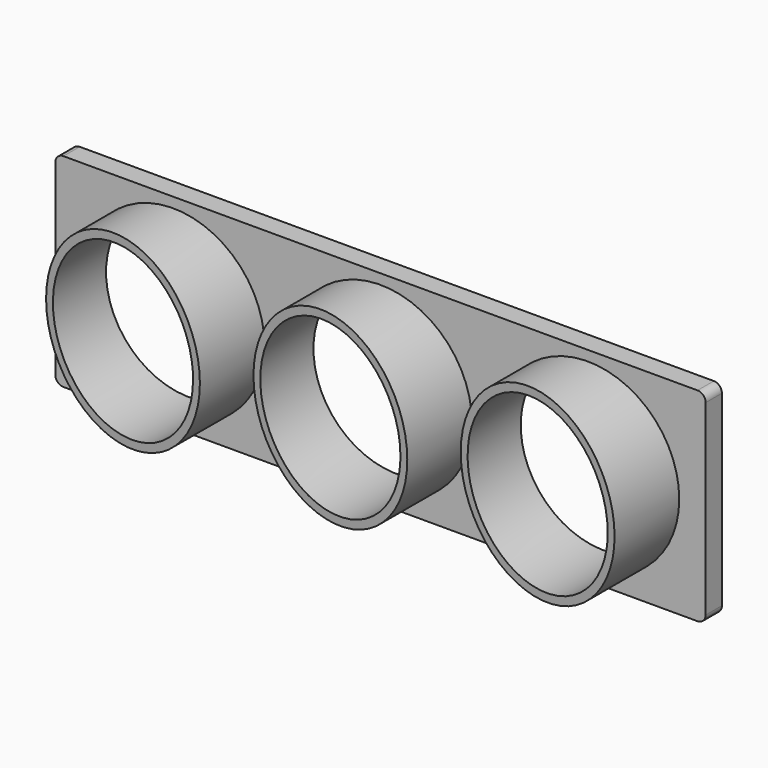
from build123d import *

# Parameters (mm, degrees)
F0_W     = 203.2
F0_H     = 63.5
F1_DEPTH = 6.35
F2_R     = 26.035
F3_DEPTH = 12.7
F4_R     = 28.575
F4_R_2   = 26.035
F5_DEPTH = 25.4
F7_DEPTH = 31.75
F8_R     = 2.54


# Not quite as in the source:
# - a feature names something its author has since deleted; it is built from what else it names


with BuildPart() as f1:
    # F0 (on Front) → F1 (new body)
    with BuildSketch(Plane.XZ):
        Rectangle(F0_W, F0_H)
    extrude(amount=F1_DEPTH)

    # F2 (on face) → F3 (cut)
    with BuildSketch(Plane.XZ.offset(6.35)):
        with Locations((-64.8028552532, 0)):
            Circle(F2_R)
        Circle(F2_R)
        with Locations((64.77, 0)):
            Circle(F2_R)
    extrude(amount=-F3_DEPTH, mode=Mode.SUBTRACT)

    # F4 (on face) → F5 (join)
    with BuildSketch(Plane.XZ.offset(6.35)):
        with Locations((-64.8028552532, 0)):
            Circle(F4_R)
        with Locations((-64.8028552532, 0)):
            Circle(F4_R_2, mode=Mode.SUBTRACT)
        Circle(F4_R)
        Circle(F4_R_2, mode=Mode.SUBTRACT)
        with Locations((64.77, 0)):
            Circle(F4_R)
        with Locations((64.77, 0)):
            Circle(F4_R_2, mode=Mode.SUBTRACT)
    extrude(amount=F5_DEPTH)

    # F6 (on Top) → F7 (cut, symmetric)
    with BuildSketch(Plane.XY):
        Polygon((35.6169715524, -20.1309207911), (35.6169715524, -32.004), (95.3069715524, -32.004), align=None)
        Polygon((-29.1554266587, -20.1309207911), (-29.1554266587, -32.004), (30.5345733413, -32.004), align=None)
        Polygon((-93.9486771822, -20.1309207911), (-93.9486771822, -32.004), (-34.2586771822, -32.004), align=None)
    extrude(amount=F7_DEPTH, both=True, mode=Mode.SUBTRACT)

    # F8
    f8_edges = [f1.edges().sort_by_distance(p)[0] for p in [
        (-101.6, -3.175, -31.75),
        (-101.6, -3.175, 31.75),
        (101.6, -3.175, 31.75),
        (101.6, -3.175, -31.75),
    ]]
    fillet(f8_edges, radius=F8_R)


solid = f1.part
